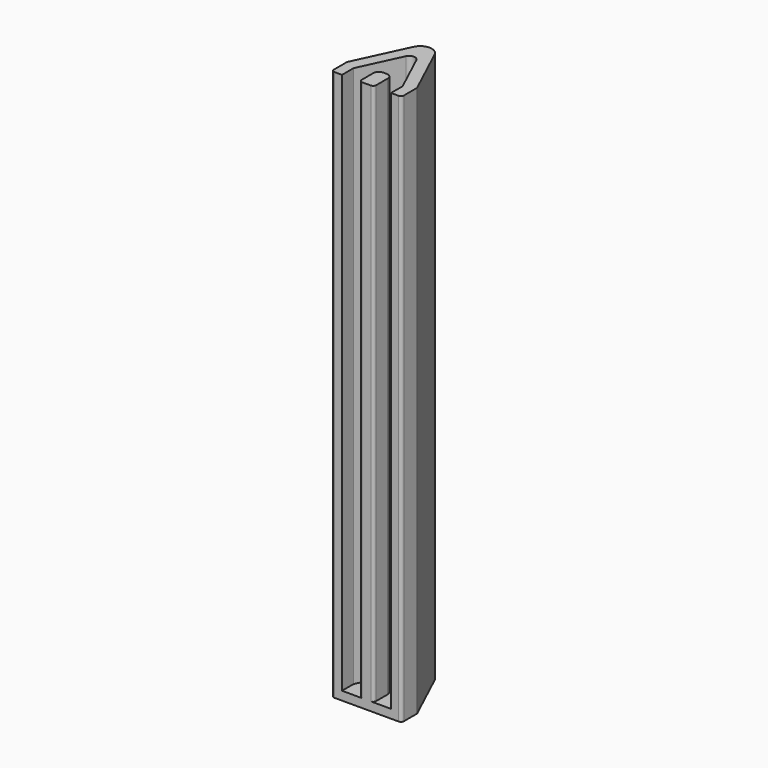
from build123d import *

# Parameters (mm, degrees)
F1_DEPTH = 1.5
F2_DEPTH = 95
F3_R     = 0.5


# Not quite as in the source:
# - a feature names something its author has since deleted; it is built from what else it names


with BuildPart() as f1:
    # F0 (on Top) → F1 (new body)
    with BuildSketch(Plane.XY):
        with BuildLine():
            ThreePointArc((0.906307787, -1.9435833214), (0, -1.3662015832), (-0.906307787, -1.9435833214))
            Line((-0.906307787, -1.9435833214), (-4.2261826174, -9.0630778704))
            Line((-4.2261826174, -9.0630778704), (-4.2261826174, -11.5630778704))
            Line((-4.2261826174, -11.5630778704), (-1.25, -11.5630778704))
            Line((-1.25, -11.5630778704), (-1.25, -8.5630778704))
            ThreePointArc((-1.25, -8.5630778704), (-0.9571067812, -7.8559710892), (-0.25, -7.5630778704))
            Line((-0.25, -7.5630778704), (0.25, -7.5630778704))
            ThreePointArc((0.25, -7.5630778704), (0.9571067812, -7.8559710892), (1.25, -8.5630778704))
            Line((1.25, -8.5630778704), (1.25, -11.5630778704))
            Line((1.25, -11.5630778704), (4.2261826174, -11.5630778704))
            Line((4.2261826174, -11.5630778704), (4.2261826174, -9.0630778704))
            Line((4.2261826174, -9.0630778704), (0.906307787, -1.9435833214))
        make_face()
        with BuildLine():
            Line((-4.2261826174, -9.0630778704), (-0.906307787, -1.9435833214))
            ThreePointArc((-0.906307787, -1.9435833214), (0, -1.3662015832), (0.906307787, -1.9435833214))
            Line((0.906307787, -1.9435833214), (4.2261826174, -9.0630778704))
            Line((4.2261826174, -9.0630778704), (4.2261826174, -11.5630778704))
            Line((4.2261826174, -11.5630778704), (6.0387981915, -11.5630778704))
            Line((6.0387981915, -11.5630778704), (6.0387981915, -8.2178413469))
            Line((6.0387981915, -8.2178413469), (1.8126155741, 0.8452365235))
            ThreePointArc((1.8126155741, 0.8452365235), (0, 2), (-1.8126155741, 0.8452365235))
            Line((-1.8126155741, 0.8452365235), (-6.0387981915, -8.2178413469))
            Line((-6.0387981915, -8.2178413469), (-6.0387981915, -11.5630778704))
            Line((-6.0387981915, -11.5630778704), (-4.2261826174, -11.5630778704))
            Line((-4.2261826174, -11.5630778704), (-4.2261826174, -9.0630778704))
        make_face()
        with BuildLine():
            Line((-1.25, -8.5630778704), (-1.25, -11.5630778704))
            Line((-1.25, -11.5630778704), (1.25, -11.5630778704))
            Line((1.25, -11.5630778704), (1.25, -8.5630778704))
            ThreePointArc((1.25, -8.5630778704), (0.9571067812, -7.8559710892), (0.25, -7.5630778704))
            Line((0.25, -7.5630778704), (-0.25, -7.5630778704))
            ThreePointArc((-0.25, -7.5630778704), (-0.9571067812, -7.8559710892), (-1.25, -8.5630778704))
        make_face()
    extrude(amount=F1_DEPTH)

    # F0 (on Top) → F2 (join)
    with BuildSketch(Plane.XY):
        with BuildLine():
            Line((-4.2261826174, -9.0630778704), (-0.906307787, -1.9435833214))
            ThreePointArc((-0.906307787, -1.9435833214), (0, -1.3662015832), (0.906307787, -1.9435833214))
            Line((0.906307787, -1.9435833214), (4.2261826174, -9.0630778704))
            Line((4.2261826174, -9.0630778704), (4.2261826174, -11.5630778704))
            Line((4.2261826174, -11.5630778704), (6.0387981915, -11.5630778704))
            Line((6.0387981915, -11.5630778704), (6.0387981915, -8.2178413469))
            Line((6.0387981915, -8.2178413469), (1.8126155741, 0.8452365235))
            ThreePointArc((1.8126155741, 0.8452365235), (0, 2), (-1.8126155741, 0.8452365235))
            Line((-1.8126155741, 0.8452365235), (-6.0387981915, -8.2178413469))
            Line((-6.0387981915, -8.2178413469), (-6.0387981915, -11.5630778704))
            Line((-6.0387981915, -11.5630778704), (-4.2261826174, -11.5630778704))
            Line((-4.2261826174, -11.5630778704), (-4.2261826174, -9.0630778704))
        make_face()
        with BuildLine():
            Line((-1.25, -8.5630778704), (-1.25, -11.5630778704))
            Line((-1.25, -11.5630778704), (1.25, -11.5630778704))
            Line((1.25, -11.5630778704), (1.25, -8.5630778704))
            ThreePointArc((1.25, -8.5630778704), (0.9571067812, -7.8559710892), (0.25, -7.5630778704))
            Line((0.25, -7.5630778704), (-0.25, -7.5630778704))
            ThreePointArc((-0.25, -7.5630778704), (-0.9571067812, -7.8559710892), (-1.25, -8.5630778704))
        make_face()
    extrude(amount=F2_DEPTH)

    # F3
    f3_edges = [f1.edges().sort_by_distance(p)[0] for p in [
        (-6.038798, -8.217841, 47.5),
        (-6.038798, -11.563078, 47.5),
        (6.038798, -8.217841, 47.5),
        (6.038798, -11.563078, 47.5),
        (-1.25, -11.563078, 48.25),
        (1.25, -11.563078, 48.25),
    ]]
    fillet(f3_edges, radius=F3_R)


solid = f1.part
